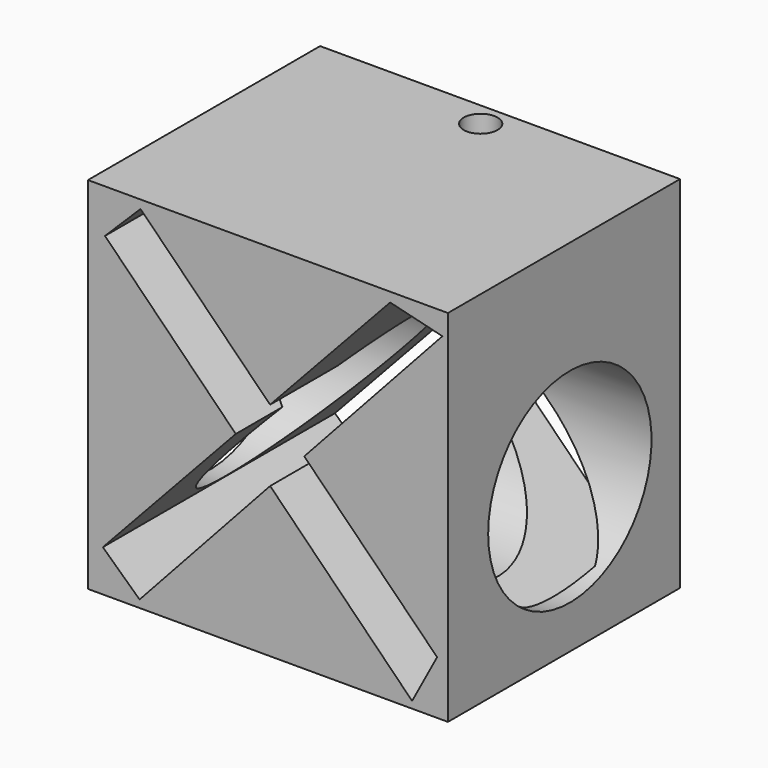
from build123d import *

# Parameters (mm, degrees)
F1_DEPTH = 54
F3_D     = 38
F5_D     = 6.3
F5_DEPTH = 12
F5_TIP   = 1.8927109499


# Not quite as in the source:
# - a feature names something its author has since deleted; it is built from what else it names


with BuildPart() as f1:
    # F0 (on Front) → F1 (new body)
    with BuildSketch(Plane.XZ):
        Polygon((28.0907023698, -33.5), (33.5, -33.5), (33.5, -25.5690795523), (31.4847062311, -23.5432559017), (26.8295921046, -32.2290576438), align=None)
        Polygon((-25.1683651974, -33.5), (28.0907023698, -33.5), (26.8295921046, -32.2290576438), (0.4087149623, -5.6021933843), (-23.8942493722, -32.1102777692), align=None)
        Polygon((31.4847062311, -23.5432559017), (33.5, -25.5690795523), (33.5, 30.4916165769), (32.4673100421, 29.3652258959), (6.7529691073, 1.3177042019), align=None)
        Polygon((-33.5, -33.5), (-25.1683651974, -33.5), (-23.8942493722, -32.1102777692), (-30.7295821389, -25.7524549578), (-33.5, -28.7309475243), align=None)
        Polygon((32.4673100421, 29.3652258959), (33.5, 30.4916165769), (33.5, 33.5), (24.3835517234, 33.5), (22.7440218852, 31.7373318104), align=None)
        Polygon((-33.5, 28.5708867013), (-33.5, -28.7309475243), (-30.7295821389, -25.7524549578), (-5.9894273378, 0.8458312449), (-30.3316890574, 25.3778744124), align=None)
        Polygon((22.7440218852, 31.7373318104), (24.3835517234, 33.5), (-25.2620486716, 33.5), (-23.714253223, 31.9441173419), (0.3945803139, 7.7093154877), align=None)
        Polygon((-33.5, 33.5), (-33.5, 28.5708867013), (-30.3316890574, 25.3778744124), (-23.714253223, 31.9441173419), (-25.2620486716, 33.5), align=None)
    extrude(amount=-F1_DEPTH)

    # F3 (through all)
    with Locations(Plane.YZ.offset(33.5)):
        with Locations((28.3605195582, -6.5)):
            Hole(F3_D / 2)

    # F5
    with Locations(Plane.XY.offset(33.5)):
        with Locations((0, 49.4885705411)):
            Hole(F5_D / 2, depth=F5_DEPTH)
            with Locations((0, 0, -(F5_DEPTH + F5_TIP / 2))):  # 118° drill point
                Cone(0, F5_D / 2, F5_TIP, mode=Mode.SUBTRACT)


solid = f1.part
